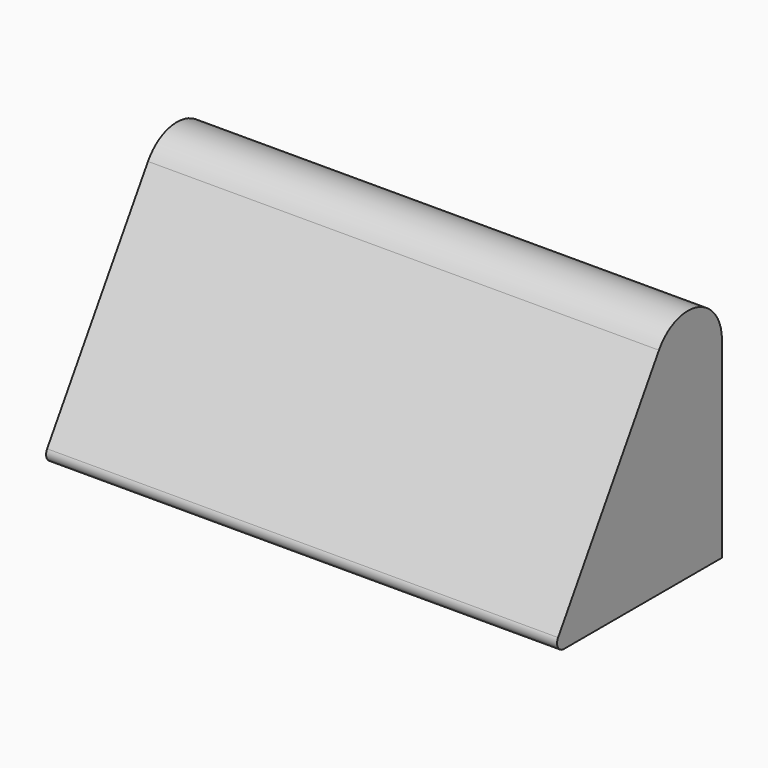
from build123d import *

# Parameters (mm, degrees)
F1_DEPTH    = 30
F3_DEPTH    = 25
F5_T1_DEPTH = 147.1699056603
F6_R        = 1


# Not quite as in the source:
# - a fillet or chamfer that OpenCascade refuses, or shapes differently, is made with other operations: its cross-section is extruded or revolved along the edge and cut away or added


with BuildPart() as f1:
    # F0 (on Right) → F1 (new body)
    with BuildSketch(Plane.YZ):
        Polygon((-25, 0), (0, 0), (0, 40), align=None)
    extrude(amount=F1_DEPTH)

    # F2 (on face) → F3 (cut)
    with BuildSketch(Plane.YZ.offset(30)):
        Polygon((-14.8754669353, 3.6356896162), (0, 3.6356896162), (0, 27.4364367127), align=None)
    extrude(amount=-F3_DEPTH, mode=Mode.SUBTRACT)

    # F4: F1 across face


with BuildPart() as f1_1:
    add(f1.part)
    add(f1.part.mirror(Plane(origin=(30, -10.1830881956, 14.3002167565), x_dir=(0, 1, 0), z_dir=(1, 0, 0))))

    # F5: fillet of radius 5 on 1 edges, made by hand

    # F5_s2 → F5_t1 (cut)
    with BuildSketch(Plane.YZ.offset(-43.5849528301)):
        with BuildLine():
            ThreePointArc((0, 22.5660188679), (-3.6215874348, 27.3722625988), (-9.23999152, 25.216013568))
            Line((-9.23999152, 25.216013568), (0, 40))
            Line((0, 40), (0, 22.5660188679))
        make_face()
    extrude(amount=F5_T1_DEPTH, mode=Mode.SUBTRACT)

    # F6
    f6_edges = [f1_1.edges().sort_by_distance(p)[0] for p in [
        (30, -25, 0),
    ]]
    fillet(f6_edges, radius=F6_R)


solid = f1_1.part
